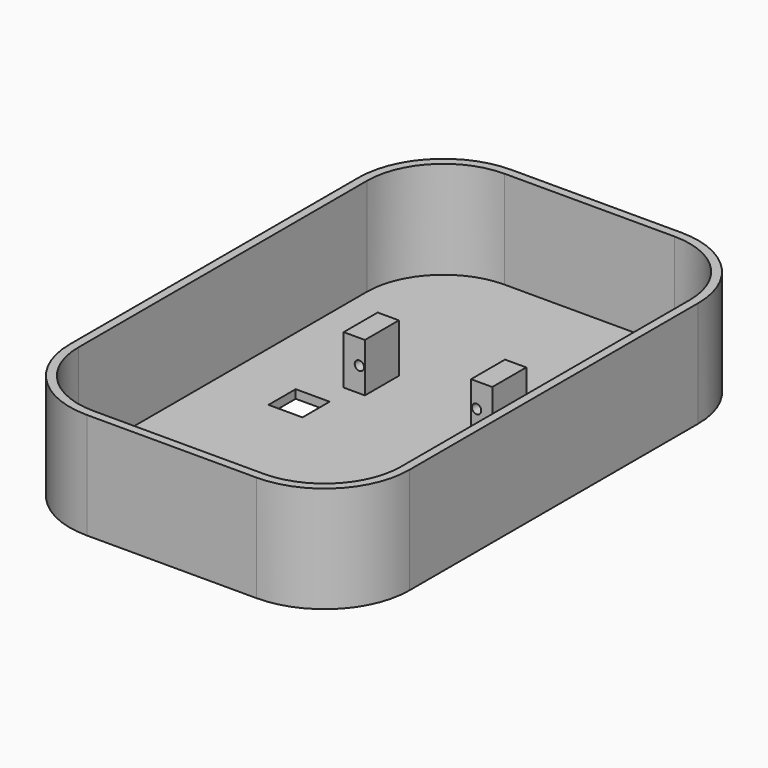
from build123d import *

# Parameters (mm, degrees)
F1_DEPTH  = 2
F2_DEPTH  = 25
F3_T      = -2
F4_W      = 8
F4_H      = 8
F5_DEPTH  = 25
F6_W      = 35
F6_H      = 11.5
F6_R      = 1.1
F7_DEPTH  = 30
F8_DEPTH  = 10
F9_W      = 25
F9_H      = 11.5
F10_DEPTH = 25
F11_DEPTH = 10


# Not quite as in the source:
# - a feature names something its author has since deleted; it is built from what else it names


with BuildPart() as f1:
    # F0 (on Top) → F1 (new body)
    with BuildSketch(Plane.XY):
        with BuildLine():
            Line((-20, -62.5), (20, -62.5))
            ThreePointArc((20, -62.5), (34.1421356237, -56.6421356237), (40, -42.5))
            Line((40, -42.5), (40, 42.5))
            ThreePointArc((40, 42.5), (34.1421356237, 56.6421356237), (20, 62.5))
            Line((20, 62.5), (-20, 62.5))
            ThreePointArc((-20, 62.5), (-34.1421356237, 56.6421356237), (-40, 42.5))
            Line((-40, 42.5), (-40, -42.5))
            ThreePointArc((-40, -42.5), (-34.1421356237, -56.6421356237), (-20, -62.5))
        make_face()
    extrude(amount=F1_DEPTH)

    # F0 (on Top) → F2 (join)
    with BuildSketch(Plane.XY):
        with BuildLine():
            Line((-20, -62.5), (20, -62.5))
            ThreePointArc((20, -62.5), (34.1421356237, -56.6421356237), (40, -42.5))
            Line((40, -42.5), (40, 42.5))
            ThreePointArc((40, 42.5), (34.1421356237, 56.6421356237), (20, 62.5))
            Line((20, 62.5), (-20, 62.5))
            ThreePointArc((-20, 62.5), (-34.1421356237, 56.6421356237), (-40, 42.5))
            Line((-40, 42.5), (-40, -42.5))
            ThreePointArc((-40, -42.5), (-34.1421356237, -56.6421356237), (-20, -62.5))
        make_face()
    extrude(amount=F2_DEPTH)

    # F3
    f3_openings = [f1.faces().sort_by_distance(p)[0] for p in [
        (0, 0, 25),
    ]]
    offset(amount=F3_T, openings=f3_openings)

    # F4 (on face) → F5 (cut)
    with BuildSketch(Plane.XY.offset(2)):
        with Locations((20, 0)):
            Rectangle(F4_W, F4_H)
        with Locations((-20, 0)):
            Rectangle(F4_W, F4_H)
    extrude(amount=-F5_DEPTH, mode=Mode.SUBTRACT)

    # F6 (on Front) → F7 (join)
    with BuildSketch(Plane.XZ):
        with Locations((0, 7.75)):
            Rectangle(F6_W, F6_H)
        with Locations((-13.8, 7.75)):
            Circle(F6_R, mode=Mode.SUBTRACT)
        with Locations((13.8, 7.75)):
            Circle(F6_R, mode=Mode.SUBTRACT)
    extrude(amount=-F7_DEPTH)

    # F8 (cut): a face of the model
    f8_faces = [f1.faces().sort_by_distance(p)[0] for p in [
        (0, 0, 7.75),
    ]]
    extrude(f8_faces, amount=-F8_DEPTH, mode=Mode.SUBTRACT)

    # F9 (on face) → F10 (cut)
    with BuildSketch(Plane.XZ.offset(-10)):
        with Locations((0, 7.75)):
            Rectangle(F9_W, F9_H)
    extrude(amount=-F10_DEPTH, mode=Mode.SUBTRACT)

    # F11 (cut): faces of the model
    f11_faces = [f1.faces().sort_by_distance(p)[0] for p in [
        (15.0849479566, 30, 7.75),
        (-15.0849479566, 30, 7.75),
    ]]
    extrude(f11_faces, amount=-F11_DEPTH, mode=Mode.SUBTRACT)


solid = f1.part
